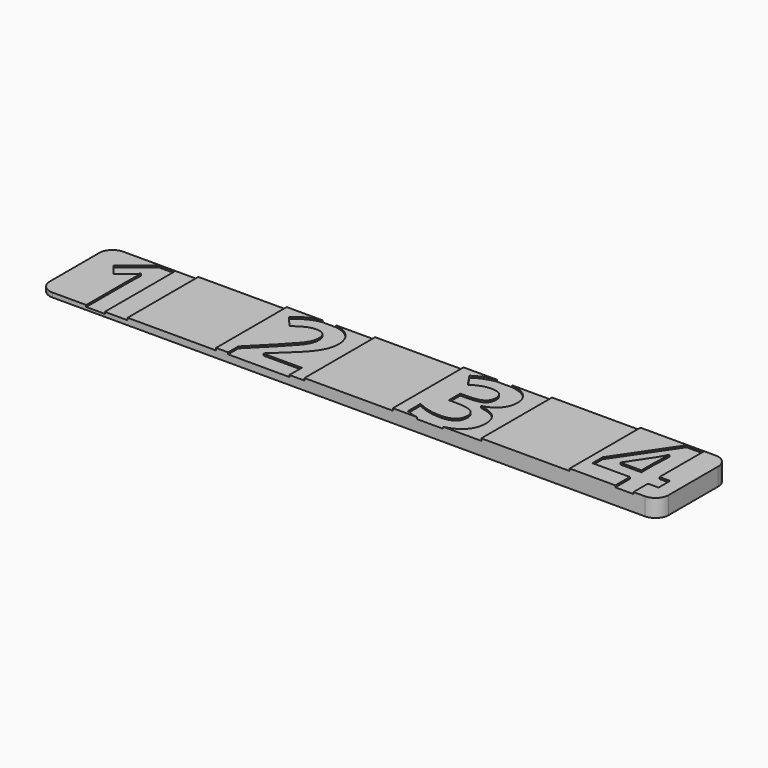
from build123d import *

# Parameters (mm, degrees)
F0_W          = 20
F0_H          = 20
F1_DEPTH      = 1
F2_DEPTH      = 1.5
F3_DEPTH      = 2
F4_DEPTH      = 2.5
F5_DEPTH      = 3
F6_DEPTH      = 3.5
F7_DEPTH      = 4
F8_TEXT_SIZE  = 27.7777777778
F11_TEXT_SIZE = 27.7777777778
F12_DEPTH     = 0.4
F13_R         = 3


# Not quite as in the source:
# - Text() gives the source's letters only with a copy of the font that has no kerning and outlines rounded to 1/6400 em; it was checked with that copy


with BuildPart() as f1:
    # F0 (on Top) → F1 (new body)
    with BuildSketch(Plane.XY):
        with Locations((-40, 0)):
            Rectangle(F0_W, F0_H)
    extrude(amount=F1_DEPTH)

    # F0 (on Top) → F2 (join)
    with BuildSketch(Plane.XY):
        with Locations((-20, 0)):
            Rectangle(F0_W, F0_H)
    extrude(amount=F2_DEPTH)

    # F0 (on Top) → F3 (join)
    with BuildSketch(Plane.XY):
        Rectangle(F0_W, F0_H)
    extrude(amount=F3_DEPTH)

    # F0 (on Top) → F4 (join)
    with BuildSketch(Plane.XY):
        with Locations((20, 0)):
            Rectangle(F0_W, F0_H)
    extrude(amount=F4_DEPTH)

    # F0 (on Top) → F5 (join)
    with BuildSketch(Plane.XY):
        with Locations((40, 0)):
            Rectangle(F0_W, F0_H)
    extrude(amount=F5_DEPTH)

    # F0 (on Top) → F6 (join)
    with BuildSketch(Plane.XY):
        with Locations((60, 0)):
            Rectangle(F0_W, F0_H)
    extrude(amount=F6_DEPTH)

    # F0 (on Top) → F7 (join)
    with BuildSketch(Plane.XY):
        with Locations((80, 0)):
            Rectangle(F0_W, F0_H)
    extrude(amount=F7_DEPTH)

    # F8 (on face) + F10 (on face) + F9 (on face) + F11 (on face) → F12 (cut)
    with BuildSketch(Plane.XY.offset(1)):
        with Locations((-46.6384548611, -10)):
            Text('1', F8_TEXT_SIZE, font='Open Sans', font_style=FontStyle.BOLD, text_align=(TextAlign.LEFT, TextAlign.BOTTOM))
    with BuildSketch(Plane.XY.offset(3)):
        with BuildLine():
            add(Edge.make_bspline(
                [(45.9092881944, 5.3949652778), (45.9092881944, 3.5373263889), (44.7829861111, 2.2352430556)],
                knots=[0, 0, 0, 1, 1, 1], degree=2))
            add(Edge.make_bspline(
                [(44.1254340278, 8.8650173611), (45.9092881944, 7.6171875), (45.9092881944, 5.3949652778)],
                knots=[0, 0, 0, 1, 1, 1], degree=2))
            add(Edge.make_bspline(
                [(40.9981629037, 10), (42.8780272016, 9.7375951288), (44.1254340278, 8.8650173611)],
                knots=[0.3007237646, 0.3007237646, 0.3007237646, 1, 1, 1], degree=2))
            Line((40.9981629037, 10), (37.517810144, 10))
            add(Edge.make_bspline(
                [(32.79296875, 8.1597222222), (34.8535967745, 9.6433743999), (37.517810144, 10)],
                knots=[0, 0, 0, 0.759629915, 0.759629915, 0.759629915], degree=2))
            Line((32.79296875, 8.1597222222), (34.7330729167, 5.2734375))
            add(Edge.make_bspline(
                [(36.9769965278, 6.3975694444), (35.9657118056, 6.0720486111), (34.7330729167, 5.2734375)],
                knots=[0, 0, 0, 1, 1, 1], degree=2))
            add(Edge.make_bspline(
                [(38.96484375, 6.7230902778), (37.98828125, 6.7230902778), (36.9769965278, 6.3975694444)],
                knots=[0, 0, 0, 1, 1, 1], degree=2))
            add(Edge.make_bspline(
                [(41.7860243056, 4.4704861111), (41.7860243056, 6.7230902778), (38.96484375, 6.7230902778)],
                knots=[0, 0, 0, 1, 1, 1], degree=2))
            add(Edge.make_bspline(
                [(40.7204861111, 2.4045138889), (41.7860243056, 3.0078125), (41.7860243056, 4.4704861111)],
                knots=[0, 0, 0, 1, 1, 1], degree=2))
            add(Edge.make_bspline(
                [(37.3502604167, 1.8012152778), (39.6549479167, 1.8012152778), (40.7204861111, 2.4045138889)],
                knots=[0, 0, 0, 1, 1, 1], degree=2))
            Line((37.3502604167, 1.8012152778), (35.8181423611, 1.8012152778))
            Line((35.8181423611, 1.8012152778), (35.8181423611, -1.4149305556))
            Line((35.8181423611, -1.4149305556), (37.32421875, -1.4149305556))
            add(Edge.make_bspline(
                [(40.9592013889, -1.9986979167), (39.8198784722, -1.4149305556), (37.32421875, -1.4149305556)],
                knots=[0, 0, 0, 1, 1, 1], degree=2))
            add(Edge.make_bspline(
                [(42.0985243056, -3.9756944444), (42.0985243056, -2.5824652778), (40.9592013889, -1.9986979167)],
                knots=[0, 0, 0, 1, 1, 1], degree=2))
            add(Edge.make_bspline(
                [(41.1089409722, -6.2434895833), (42.0985243056, -5.5381944444), (42.0985243056, -3.9756944444)],
                knots=[0, 0, 0, 1, 1, 1], degree=2))
            add(Edge.make_bspline(
                [(38.0403645833, -6.9487847222), (40.1193576389, -6.9487847222), (41.1089409722, -6.2434895833)],
                knots=[0, 0, 0, 1, 1, 1], degree=2))
            add(Edge.make_bspline(
                [(35.3016493056, -6.58203125), (36.6861979167, -6.9487847222), (38.0403645833, -6.9487847222)],
                knots=[0, 0, 0, 1, 1, 1], degree=2))
            add(Edge.make_bspline(
                [(32.7669270833, -5.6336805556), (33.9171006944, -6.2152777778), (35.3016493056, -6.58203125)],
                knots=[0, 0, 0, 1, 1, 1], degree=2))
            Line((32.7669270833, -5.6336805556), (32.7669270833, -9.2013888889))
            add(Edge.make_bspline(
                [(35.4171554992, -10), (34.002190365, -9.732015029), (32.7669270833, -9.2013888889)],
                knots=[0.5050353738, 0.5050353738, 0.5050353738, 1, 1, 1], degree=2))
            Line((35.4171554992, -10), (41.3753971165, -10))
            add(Edge.make_bspline(
                [(44.4162326389, -8.6783854167), (43.2005677188, -9.6130231952), (41.3753971165, -10)],
                knots=[0, 0, 0, 0.5859606644, 0.5859606644, 0.5859606644], degree=2))
            add(Edge.make_bspline(
                [(46.4908854167, -4.2230902778), (46.4908854167, -7.0833333333), (44.4162326389, -8.6783854167)],
                knots=[0, 0, 0, 1, 1, 1], degree=2))
            add(Edge.make_bspline(
                [(45.2582465278, -1.0959201389), (46.4908854167, -2.2569444444), (46.4908854167, -4.2230902778)],
                knots=[0, 0, 0, 1, 1, 1], degree=2))
            add(Edge.make_bspline(
                [(41.62109375, 0.3645833333), (44.0256076389, 0.0651041667), (45.2582465278, -1.0959201389)],
                knots=[0, 0, 0, 1, 1, 1], degree=2))
            Line((41.62109375, 0.3645833333), (41.62109375, 0.4427083333))
            add(Edge.make_bspline(
                [(44.7829861111, 2.2352430556), (43.6566840278, 0.9331597222), (41.62109375, 0.4427083333)],
                knots=[0, 0, 0, 1, 1, 1], degree=2))
        make_face()
    with BuildSketch(Plane.XY.offset(2)):
        with BuildLine():
            Line((-7.2764756944, -10), (6.5863715278, -10))
            Line((6.5863715278, -10), (6.5863715278, -6.4713541667))
            Line((6.5863715278, -6.4713541667), (-2.0551215278, -6.4713541667))
            Line((-2.0551215278, -6.4713541667), (-2.0551215278, -6.2847222222))
            Line((-2.0551215278, -6.2847222222), (0.4969618056, -3.8845486111))
            add(Edge.make_bspline(
                [(4.0559895833, -0.2886284722), (3.0447048611, -1.5494791667), (0.4969618056, -3.8845486111)],
                knots=[0, 0, 0, 1, 1, 1], degree=2))
            add(Edge.make_bspline(
                [(5.5490451389, 2.1723090278), (5.0672743056, 0.9722222222), (4.0559895833, -0.2886284722)],
                knots=[0, 0, 0, 1, 1, 1], degree=2))
            add(Edge.make_bspline(
                [(6.0308159722, 4.7439236111), (6.0308159722, 3.3723958333), (5.5490451389, 2.1723090278)],
                knots=[0, 0, 0, 1, 1, 1], degree=2))
            add(Edge.make_bspline(
                [(5.2430555556, 7.5368923611), (6.0308159722, 6.3151041667), (6.0308159722, 4.7439236111)],
                knots=[0, 0, 0, 1, 1, 1], degree=2))
            add(Edge.make_bspline(
                [(3.0316840278, 9.4357638889), (4.4552951389, 8.7586805556), (5.2430555556, 7.5368923611)],
                knots=[0, 0, 0, 1, 1, 1], degree=2))
            add(Edge.make_bspline(
                [(1.1948518662, 10), (2.1892597191, 9.8364291089), (3.0316840278, 9.4357638889)],
                knots=[0.4082482905, 0.4082482905, 0.4082482905, 1, 1, 1], degree=2))
            Line((1.1948518662, 10), (-1.9375204448, 10))
            add(Edge.make_bspline(
                [(-2.7994791667, 9.8350694444), (-2.386334973, 9.9357979336), (-1.9375204448, 10)],
                knots=[0, 0, 0, 0.3626225608, 0.3626225608, 0.3626225608], degree=2))
            add(Edge.make_bspline(
                [(-4.90234375, 9.04296875), (-3.9388020833, 9.5572916667), (-2.7994791667, 9.8350694444)],
                knots=[0, 0, 0, 1, 1, 1], degree=2))
            add(Edge.make_bspline(
                [(-7.3285590278, 7.2786458333), (-5.8658854167, 8.5286458333), (-4.90234375, 9.04296875)],
                knots=[0, 0, 0, 1, 1, 1], degree=2))
            Line((-7.3285590278, 7.2786458333), (-5.0499131944, 4.5789930556))
            add(Edge.make_bspline(
                [(-2.7842881944, 6.0850694444), (-3.8693576389, 5.5555555556), (-5.0499131944, 4.5789930556)],
                knots=[0, 0, 0, 1, 1, 1], degree=2))
            add(Edge.make_bspline(
                [(-0.5490451389, 6.6145833333), (-1.69921875, 6.6145833333), (-2.7842881944, 6.0850694444)],
                knots=[0, 0, 0, 1, 1, 1], degree=2))
            add(Edge.make_bspline(
                [(1.2087673611, 6.0308159722), (0.5490451389, 6.6145833333), (-0.5490451389, 6.6145833333)],
                knots=[0, 0, 0, 1, 1, 1], degree=2))
            add(Edge.make_bspline(
                [(1.8684895833, 4.2534722222), (1.8684895833, 5.4470486111), (1.2087673611, 6.0308159722)],
                knots=[0, 0, 0, 1, 1, 1], degree=2))
            add(Edge.make_bspline(
                [(1.5690104167, 2.7083333333), (1.8684895833, 3.4548611111), (1.8684895833, 4.2534722222)],
                knots=[0, 0, 0, 1, 1, 1], degree=2))
            add(Edge.make_bspline(
                [(0.5924479167, 1.0872395833), (1.26953125, 1.9618055556), (1.5690104167, 2.7083333333)],
                knots=[0, 0, 0, 1, 1, 1], degree=2))
            add(Edge.make_bspline(
                [(-2.2981770833, -2.0529513889), (-0.0846354167, 0.2126736111), (0.5924479167, 1.0872395833)],
                knots=[0, 0, 0, 1, 1, 1], degree=2))
            Line((-2.2981770833, -2.0529513889), (-7.2764756944, -7.0833333333))
            Line((-7.2764756944, -7.0833333333), (-7.2764756944, -10))
        make_face()
    with BuildSketch(Plane.XY.offset(4)):
        with Locations((71.3888888889, -10)):
            Text('4', F11_TEXT_SIZE, font='Open Sans', font_style=FontStyle.BOLD, text_align=(TextAlign.LEFT, TextAlign.BOTTOM))
    extrude(amount=-F12_DEPTH, mode=Mode.SUBTRACT)

    # F13
    f13_edges = [f1.edges().sort_by_distance(p)[0] for p in [
        (90, -10, 2),
        (90, 10, 2),
        (-50, 10, 0.5),
        (-50, -10, 0.5),
    ]]
    fillet(f13_edges, radius=F13_R)


solid = f1.part
